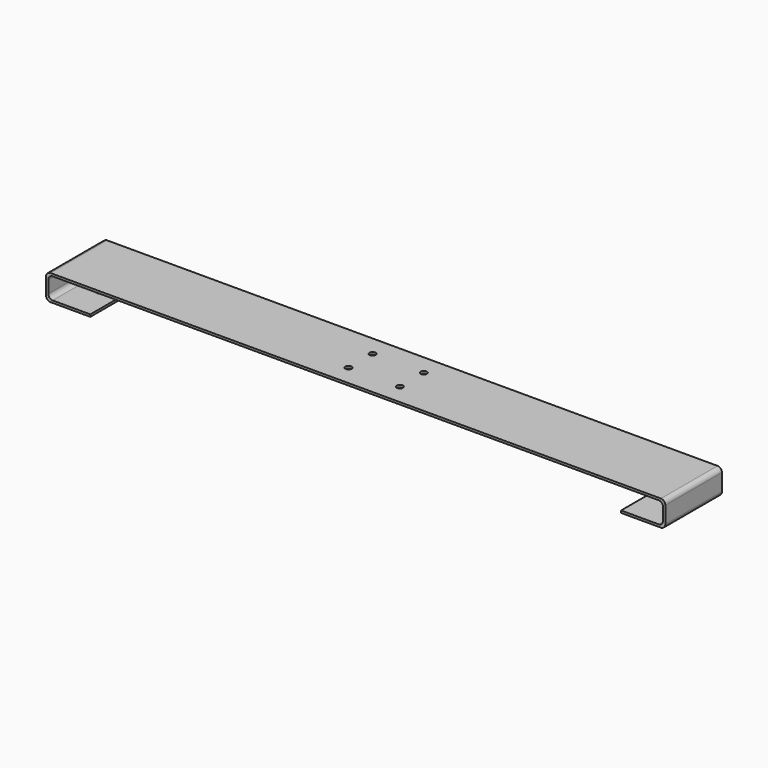
from build123d import *

# Parameters (mm, degrees)
F1_DEPTH = 40
F4_D     = 9
F4_DEPTH = 12
F4_TIP   = 2.7038727856
F5_D     = 9
F5_DEPTH = 12
F5_TIP   = 2.7038727856
F7_D     = 7
F8_R     = 5


# Not quite as in the source:
# - a feature names something its author has since deleted; it is built from what else it names


with BuildPart() as f1:
    # F0 (on Front) → F1 (new body, symmetric)
    with BuildSketch(Plane.XZ):
        Polygon((0, 29), (0, 0), (50, 0), (50, 2.5), (2.5, 2.5), (2.5, 26.5), (697.5, 26.5), (697.5, 2.5), (650, 2.5), (650, 0), (700, 0), (700, 29), align=None)
    extrude(amount=F1_DEPTH, both=True)

    # F4 (one way)
    with BuildSketch(Plane.XY.offset(2.5)):
        with Locations((670, 0)):
            Circle(F4_D / 2)
    extrude(amount=-F4_DEPTH, mode=Mode.SUBTRACT)
    with Locations(Plane.XY.offset(2.5)):
        with Locations((670, 0)):
            with Locations((0, 0, -(F4_DEPTH + F4_TIP / 2))):  # 118° drill point
                Cone(0, F4_D / 2, F4_TIP, mode=Mode.SUBTRACT)

    # F5 (one way)
    with BuildSketch(Plane.XY.offset(2.5)):
        with Locations((30, 0)):
            Circle(F5_D / 2)
    extrude(amount=-F5_DEPTH, mode=Mode.SUBTRACT)
    with Locations(Plane.XY.offset(2.5)):
        with Locations((30, 0)):
            with Locations((0, 0, -(F5_DEPTH + F5_TIP / 2))):  # 118° drill point
                Cone(0, F5_D / 2, F5_TIP, mode=Mode.SUBTRACT)

    # F7 (through all)
    with Locations(Plane(origin=(0, 0, 26.5), x_dir=(1, 0, 0), z_dir=(0, 0, -1))):
        with Locations((381.5, -17), (323.5, -17), (323.5, 17), (381.5, 17)):
            Hole(F7_D / 2)

    # F8
    f8_edges = [f1.edges().sort_by_distance(p)[0] for p in [
        (0, 0, 29),
        (0, 0, 0),
        (700, 0, 29),
        (700, 0, 0),
        (2.5, 0, 2.5),
        (2.5, 0, 26.5),
        (697.5, 0, 2.5),
        (697.5, 0, 26.5),
    ]]
    fillet(f8_edges, radius=F8_R)


solid = f1.part
